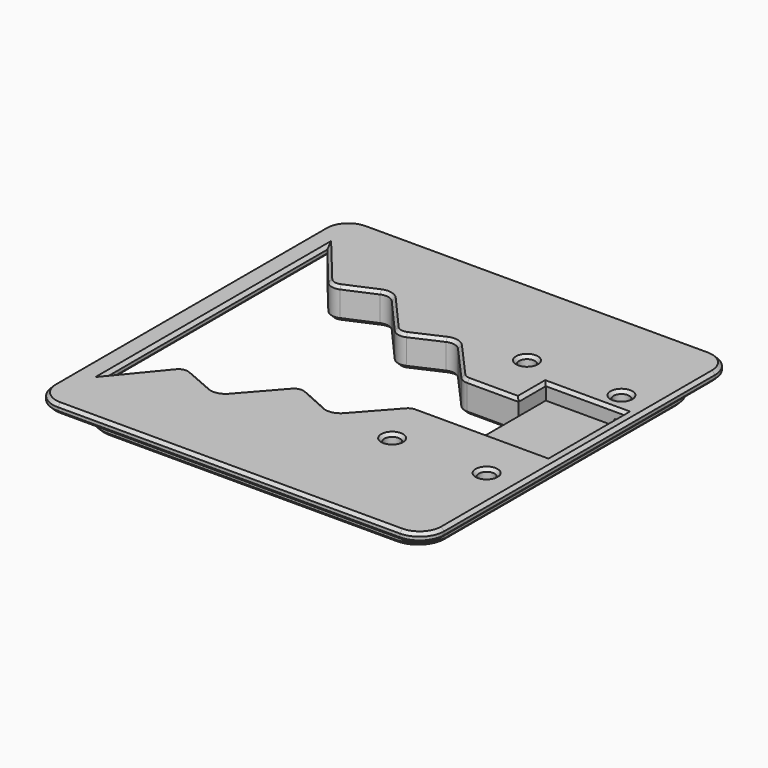
from build123d import *

# Parameters (mm, degrees)
F15_DEPTH = 2.8194
F1_W      = 50.4952
F1_H      = 50.038
F2_DEPTH  = 1.2192
F3_R      = 1.016
F4_DEPTH  = 3.175
F5_W      = 25.5439807123
F5_H      = 7.9756
F6_DEPTH  = 4.0396
F7_W      = 10.16
F7_H      = 12.3698
F8_DEPTH  = 2.032
F9_R      = 3.81
F10_R     = 3.175
F11_R     = 1.5875
F12_SIZE  = 0.396875
F13_SIZE  = 0.396875


# Not quite as in the source:
# - a feature of the source that left no trace in its solid (it failed there, or was rolled back) is left out


with BuildPart() as f15:
    # F0 (on Top) → F15 (new body)
    with BuildSketch(Plane.XY):
        Polygon((30.4991698359, 9.5009198412), (-14.2048301641, 9.5009198412), (-14.2048301641, 5.0559198412), (-8.8708301641, -1.4210801588), (-2.8619992453, 1.1873513896), (2.9147698359, -5.378930905), (8.8075698359, -2.7315337496), (14.7003698359, -9.3367816513), (21.6091698359, -9.3367816513), (21.6091698359, -16.3653786662), (14.7003698359, -16.3653786662), (8.8075698359, -22.970626568), (2.9147698359, -20.3232294125), (-2.8619992453, -26.8895117072), (-8.8708301641, -24.2810801588), (-14.2048301641, -30.7580801588), (-14.2048301641, -35.2030801588), (30.4991698359, -35.2030801588), align=None)
    extrude(amount=F15_DEPTH)

    # F1 (on face) → F2 (join)
    with BuildSketch(Plane.XY.offset(2.8194)):
        with Locations((8.1471698359, -13.7400801588)):
            Rectangle(F1_W, F1_H)
        Polygon((-8.8708301641, -24.2810801588), (-14.2048301641, -30.7580801588), (-14.2048301641, 5.0559198412), (-8.8708301641, -1.4210801588), (-2.8619992453, 1.1873513896), (2.9147698359, -5.378930905), (8.8075698359, -2.7315337496), (14.7003698359, -9.3367816513), (21.6091698359, -9.3367816513), (21.6091698359, -16.3653786662), (14.7003698359, -16.3653786662), (8.8075698359, -22.970626568), (2.9147698359, -20.3232294125), (-2.8619992453, -26.8895117072), align=None, mode=Mode.SUBTRACT)
    extrude(amount=F2_DEPTH)

    # F3 (on face) → F4 (cut)
    with BuildSketch(Plane.XY.offset(4.0386)):
        with Locations((29.2672698359, -1.8401801588)):
            Circle(F3_R)
        with Locations((29.2672698359, -23.5825801588)):
            Circle(F3_R)
        with Locations((17.0752698359, -1.8401801588)):
            Circle(F3_R)
        with Locations((17.0752698359, -23.5825801588)):
            Circle(F3_R)
    extrude(amount=-F4_DEPTH, mode=Mode.SUBTRACT)

    # F5 (on face) → F6 (cut, through all)
    with BuildSketch(Plane(origin=(0, 0, 0), x_dir=(1, 0, 0), z_dir=(0, 0, -1))):
        with Locations((8.8371794797, 12.8510801588)):
            Rectangle(F5_W, F5_H)
    extrude(amount=-F6_DEPTH, mode=Mode.SUBTRACT)

    # F7 (on face) → F8 (cut)
    with BuildSketch(Plane.XY.offset(4.0386)):
        with Locations((26.6891698359, -10.6539801588)):
            Rectangle(F7_W, F7_H)
    extrude(amount=-F8_DEPTH, mode=Mode.SUBTRACT)

    # F9
    f9_edges = [f15.edges().sort_by_distance(p)[0] for p in [
        (-14.20483, -35.20308, 1.4097),
        (30.49917, -35.20308, 1.4097),
        (30.49917, 9.50092, 1.4097),
        (-14.20483, 9.50092, 1.4097),
    ]]
    fillet(f9_edges, radius=F9_R)

    # F10
    f10_edges = [f15.edges().sort_by_distance(p)[0] for p in [
        (33.39477, -38.75908, 3.429),
        (33.39477, 11.27892, 3.429),
        (-17.10043, 11.27892, 3.429),
        (-17.10043, -38.75908, 3.429),
    ]]
    fillet(f10_edges, radius=F10_R)

    # F11
    f11_edges = [f15.edges().sort_by_distance(p)[0] for p in [
        (-8.87083, -24.28108, 2.0193),
        (2.91477, -20.323229, 2.0193),
        (14.277941, -16.83888, 2.0193),
        (14.277941, -8.86328, 2.0193),
        (8.80757, -2.731534, 2.0193),
        (-2.861999, 1.187351, 2.0193),
        (-8.87083, -1.42108, 2.0193),
        (2.91477, -5.378931, 2.0193),
        (-2.861999, -26.889512, 2.0193),
        (8.80757, -22.970627, 2.0193),
    ]]
    fillet(f11_edges, radius=F11_R)

    # F12
    f12_edges = [f15.edges().sort_by_distance(p)[0] for p in [
        (-11.918021, -27.98124, 0),
        (-8.777201, -24.670149, 0),
        (-14.20483, -31.07558, 0),
        (-5.848035, -25.593275, 0),
        (-13.088907, -34.087157, 0),
        (-2.944073, -26.522248, 0),
        (8.14717, -35.20308, 0),
        (0.021273, -23.612182, 0),
        (29.383247, -34.087157, 0),
        (2.996452, -20.69995, 0),
        (30.49917, -12.85108, 0),
        (5.865037, -21.648665, 0),
        (29.383247, 8.384997, 0),
        (8.728242, -22.598537, 0),
        (8.14717, 9.50092, 0),
        (11.693168, -19.736155, 0),
        (-13.088907, 8.384997, 0),
        (14.340089, -16.97761, 0),
        (-14.20483, 5.37342, 0),
        (18.299137, -16.83888, 0),
        (-11.918021, 2.27908, 0),
        (21.60917, -12.85108, 0),
        (-8.777201, -1.032011, 0),
        (18.299137, -8.86328, 0),
        (-5.848035, -0.108886, 0),
        (14.340089, -8.72455, 0),
        (-2.944073, 0.820088, 0),
        (11.693168, -5.966005, 0),
        (0.021273, -2.089978, 0),
        (8.728242, -3.103623, 0),
        (2.996452, -5.00221, 0),
        (5.865037, -4.053495, 0),
    ]]
    chamfer(f12_edges, length=F12_SIZE)

    # F13
    f13_edges = [f15.edges().sort_by_distance(p)[0] for p in [
        (-14.20483, -12.85108, 2.8194),
        (-17.10043, -13.74008, 2.8194),
        (8.14717, -38.75908, 2.8194),
        (33.39477, -13.74008, 2.8194),
        (8.14717, 11.27892, 2.8194),
        (23.379137, -16.83888, 4.0386),
        (14.340089, -16.97761, 4.0386),
        (31.76917, -10.65398, 4.0386),
        (11.693168, -19.736155, 4.0386),
        (26.68917, -4.46908, 4.0386),
        (8.728242, -22.598537, 4.0386),
        (21.60917, -6.66618, 4.0386),
        (5.865037, -21.648665, 4.0386),
        (18.299137, -8.86328, 4.0386),
        (2.996452, -20.69995, 4.0386),
        (14.340089, -8.72455, 4.0386),
        (0.021273, -23.612182, 4.0386),
        (11.693168, -5.966005, 4.0386),
        (-2.944073, -26.522248, 4.0386),
        (8.728242, -3.103623, 4.0386),
        (-5.848035, -25.593275, 4.0386),
        (5.865037, -4.053495, 4.0386),
        (-8.777201, -24.670149, 4.0386),
        (2.996452, -5.00221, 4.0386),
        (-11.918021, -27.98124, 4.0386),
        (0.021273, -2.089978, 4.0386),
        (-14.20483, -12.85108, 4.0386),
        (-2.944073, 0.820088, 4.0386),
        (-11.918021, 2.27908, 4.0386),
        (-5.848035, -0.108886, 4.0386),
        (-8.777201, -1.032011, 4.0386),
        (-17.10043, -13.74008, 4.0386),
        (-16.170494, 10.348984, 4.0386),
        (-16.170494, -37.829144, 4.0386),
        (8.14717, 11.27892, 4.0386),
        (8.14717, -38.75908, 4.0386),
        (32.464834, 10.348984, 4.0386),
        (32.464834, -37.829144, 4.0386),
        (33.39477, -13.74008, 4.0386),
        (16.05927, -23.58258, 4.0386),
        (28.25127, -23.58258, 4.0386),
        (16.05927, -1.84018, 4.0386),
        (28.25127, -1.84018, 4.0386),
        (-16.170494, 10.348984, 2.8194),
        (-16.170494, -37.829144, 2.8194),
        (32.464834, 10.348984, 2.8194),
        (32.464834, -37.829144, 2.8194),
    ]]
    chamfer(f13_edges, length=F13_SIZE)


solid = f15.part
